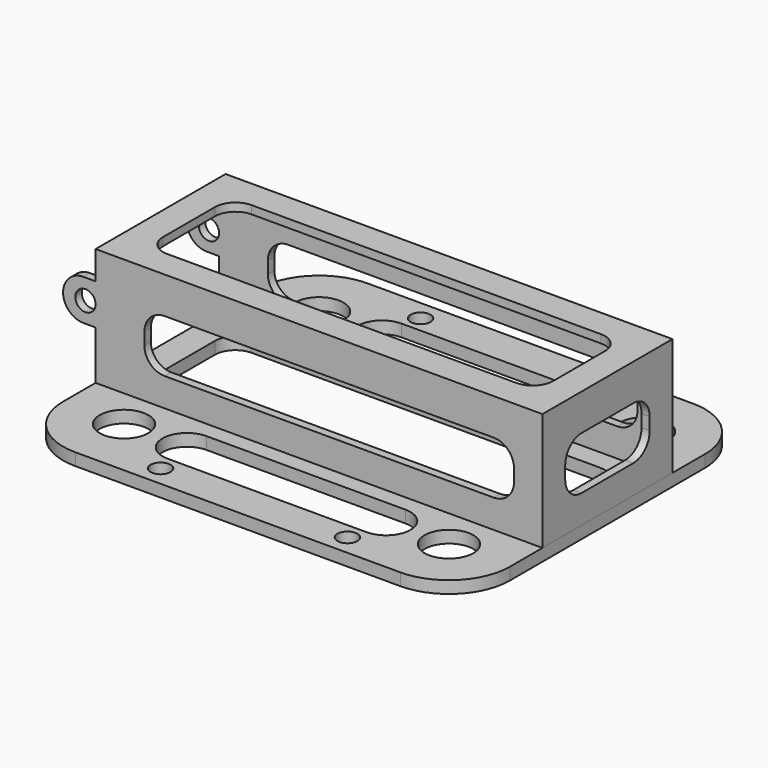
from build123d import *

# Parameters (mm, degrees)
F0_R      = 6
F0_R_2    = 2.45
F1_DEPTH  = 3
F3_DEPTH  = 27
F5_DEPTH  = 25
F7_DEPTH  = 100
F8_W      = 110
F8_H      = 40
F9_DEPTH  = 2
F11_DEPTH = 50
F12_W     = 2
F12_H     = 10
F13_DEPTH = 8
F14_R     = 2.5
F15_DEPTH = 50
F16_R     = 4.99999


# Not quite as in the source:
# - a fillet or chamfer is up to 0.001 mm smaller than in the source, because OpenCascade refuses the exact size


with BuildPart() as f1:
    # F0 (on Top) → F1 (new body)
    with BuildSketch(Plane.XY):
        with BuildLine():
            Line((36.0161362187, 47.167300203), (-43.0098088973, 47.167300203))
            ThreePointArc((-43.0098088973, 47.167300203), (-53.9298270028, 42.9526252844), (-58.4968363393, 32.1752088122))
            Line((-58.4968363393, 32.1752088122), (-58.4968363393, -27.832699797))
            ThreePointArc((-58.4968363393, -27.832699797), (-54.1034380571, -38.4393015148), (-43.4968363393, -42.832699797))
            Line((-43.4968363393, -42.832699797), (36.5031636607, -42.832699797))
            ThreePointArc((36.5031636607, -42.832699797), (47.1097653785, -38.4393015148), (51.5031636607, -27.832699797))
            Line((51.5031636607, -27.832699797), (51.5031636607, 32.1752088122))
            ThreePointArc((51.5031636607, 32.1752088122), (46.9361543242, 42.9526252844), (36.0161362187, 47.167300203))
        make_face()
        with Locations((-43.4968363393, -27.832699797)):
            Circle(F0_R, mode=Mode.SUBTRACT)
        with Locations((-26.4968363393, -37.832699797)):
            Circle(F0_R_2, mode=Mode.SUBTRACT)
        with BuildLine():
            ThreePointArc((-28.0098088973, -33.832699797), (-34.0098088973, -27.832699797), (-28.0098088973, -21.832699797))
            Line((-28.0098088973, -21.832699797), (21.0161362187, -21.832699797))
            ThreePointArc((21.0161362187, -21.832699797), (27.0161362187, -27.832699797), (21.0161362187, -33.832699797))
            Line((21.0161362187, -33.832699797), (-28.0098088973, -33.832699797))
        make_face(mode=Mode.SUBTRACT)
        with Locations((19.5031636607, -37.832699797)):
            Circle(F0_R_2, mode=Mode.SUBTRACT)
        with Locations((36.5031636607, -27.832699797)):
            Circle(F0_R, mode=Mode.SUBTRACT)
        with Locations((-43.4968363393, 32.1752088122)):
            Circle(F0_R, mode=Mode.SUBTRACT)
        with BuildLine():
            ThreePointArc((-28.0098088973, 26.1752088122), (-34.0098088973, 32.1752088122), (-28.0098088973, 38.1752088122))
            Line((-28.0098088973, 38.1752088122), (21.0161362187, 38.1752088122))
            ThreePointArc((21.0161362187, 38.1752088122), (27.0161362187, 32.1752088122), (21.0161362187, 26.1752088122))
            Line((21.0161362187, 26.1752088122), (-28.0098088973, 26.1752088122))
        make_face(mode=Mode.SUBTRACT)
        with Locations((-26.4968363393, 42.167300203)):
            Circle(F0_R_2, mode=Mode.SUBTRACT)
        with Locations((19.5031636607, 42.167300203)):
            Circle(F0_R_2, mode=Mode.SUBTRACT)
        with Locations((36.5031636607, 32.1752088122)):
            Circle(F0_R, mode=Mode.SUBTRACT)
    extrude(amount=F1_DEPTH)


with BuildPart() as f3:
    # F2 (on face) → F3 (new body)
    with BuildSketch(Plane.XY.offset(3)):
        Polygon((-58.4968363393, 22.1712545076), (-58.4968363393, 20.1712545076), (49.5031636607, 20.1712545076), (49.5031636607, -15.8287454924), (-58.4968363393, -15.8287454924), (-58.4968363393, -17.8287454924), (51.5031636607, -17.8287454924), (51.5031636607, -15.8287454924), (51.5031636607, 20.1712545076), (51.5031636607, 22.1712545076), align=None)
    extrude(amount=F3_DEPTH)

    # F4 (on face) → F5 (cut)
    with BuildSketch(Plane.YZ.offset(51.5031636607)):
        with BuildLine():
            Line((10.1712545076, 23), (-5.8287454924, 23))
            ThreePointArc((-5.8287454924, 23), (-9.3642793983, 21.5355339059), (-10.8287454924, 18))
            Line((-10.8287454924, 18), (-10.8287454924, 15))
            ThreePointArc((-10.8287454924, 15), (-9.3642793983, 11.4644660941), (-5.8287454924, 10))
            Line((-5.8287454924, 10), (10.1712545076, 10))
            ThreePointArc((10.1712545076, 10), (13.7067884136, 11.4644660941), (15.1712545076, 15))
            Line((15.1712545076, 15), (15.1712545076, 18))
            ThreePointArc((15.1712545076, 18), (13.7067884136, 21.5355339059), (10.1712545076, 23))
        make_face()
    extrude(amount=-F5_DEPTH, mode=Mode.SUBTRACT)

    # F6 (on face) → F7 (cut)
    with BuildSketch(Plane(origin=(0, 22.1712545076, 0), x_dir=(-1, 0, 0), z_dir=(0, 1, 0))):
        with BuildLine():
            Line((41.4968363393, 23), (-39.5031636607, 23))
            ThreePointArc((-39.5031636607, 23), (-43.0386975666, 21.5355339059), (-44.5031636607, 18))
            Line((-44.5031636607, 18), (-44.5031636607, 15))
            ThreePointArc((-44.5031636607, 15), (-43.0386975666, 11.4644660941), (-39.5031636607, 10))
            Line((-39.5031636607, 10), (41.4968363393, 10))
            ThreePointArc((41.4968363393, 10), (45.0323702452, 11.4644660941), (46.4968363393, 15))
            Line((46.4968363393, 15), (46.4968363393, 18))
            ThreePointArc((46.4968363393, 18), (45.0323702452, 21.5355339059), (41.4968363393, 23))
        make_face()
    extrude(amount=-F7_DEPTH, mode=Mode.SUBTRACT)

    # F8 (on face) → F9 (join)
    with BuildSketch(Plane.XY.offset(30)):
        with Locations((-3.4968363393, 2.1712545076)):
            Rectangle(F8_W, F8_H)
    extrude(amount=F9_DEPTH)


with BuildPart() as f11_tool:
    # F10 (on face) → F11 (new body)
    with BuildSketch(Plane.XY.offset(32)):
        with BuildLine():
            Line((39.5031636607, 15.1712545076), (-46.4968363393, 15.1712545076))
            ThreePointArc((-46.4968363393, 15.1712545076), (-50.0323702452, 13.7067884136), (-51.4968363393, 10.1712545076))
            Line((-51.4968363393, 10.1712545076), (-51.4968363393, -5.8287454924))
            ThreePointArc((-51.4968363393, -5.8287454924), (-50.0323702452, -9.3642793983), (-46.4968363393, -10.8287454924))
            Line((-46.4968363393, -10.8287454924), (39.5031636607, -10.8287454924))
            ThreePointArc((39.5031636607, -10.8287454924), (43.0386975666, -9.3642793983), (44.5031636607, -5.8287454924))
            Line((44.5031636607, -5.8287454924), (44.5031636607, 10.1712545076))
            ThreePointArc((44.5031636607, 10.1712545076), (43.0386975666, 13.7067884136), (39.5031636607, 15.1712545076))
        make_face()
    extrude(amount=-F11_DEPTH)


with BuildPart() as f1_1:
    add(f1.part)

    # F11: cut by f11_tool
    add(f11_tool.part, mode=Mode.SUBTRACT)


with BuildPart() as f3_1:
    add(f3.part)

    # F11: cut by f11_tool
    add(f11_tool.part, mode=Mode.SUBTRACT)

    # F12 (on face) → F13 (join)
    with BuildSketch(Plane(origin=(-58.4968363393, 0, 0), x_dir=(0, -1, 0), z_dir=(-1, 0, 0))):
        with Locations((-21.1712545076, 20)):
            Rectangle(F12_W, F12_H)
        with Locations((16.8287454924, 20)):
            Rectangle(F12_W, F12_H)
    extrude(amount=F13_DEPTH)

    # F14 (on face) → F15 (cut)
    with BuildSketch(Plane(origin=(0, 22.1712545076, 0), x_dir=(-1, 0, 0), z_dir=(0, 1, 0))):
        with Locations((60.9968363393, 20)):
            Circle(F14_R)
    extrude(amount=-F15_DEPTH, mode=Mode.SUBTRACT)

    # F16 (radius 5 in the source; OpenCascade refuses exactly that, so slightly less here)
    f16_edges = [f3_1.edges().sort_by_distance(p)[0] for p in [
        (-66.496836, -16.828745, 25),
        (-66.496836, -16.828745, 15),
        (-66.496836, 21.171255, 15),
        (-66.496836, 21.171255, 25),
    ]]
    fillet(f16_edges, radius=F16_R)


solid = Compound([f1_1.part, f3_1.part])
